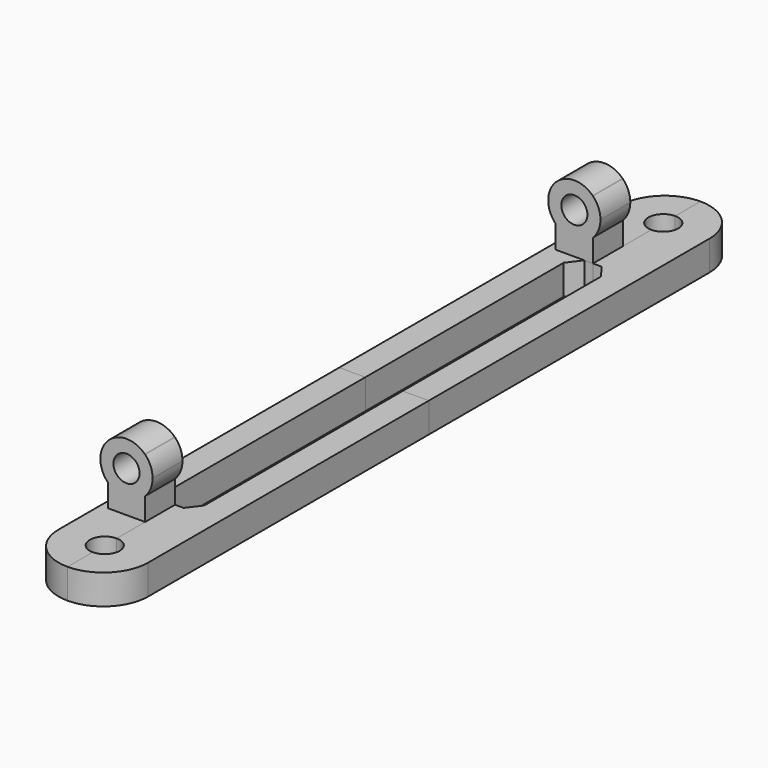
from build123d import *

# Parameters (mm, degrees)
F1_DEPTH = 4
F3_START = -35
F2_R     = 1.75
F3_DEPTH = 5
F6_R     = 5.99999
F6_2_R   = 5.99999
F6_3_R   = 5.99999
F6_4_R   = 5.99999


# Not quite as in the source:
# - a fillet or chamfer is up to 0.001 mm smaller than in the source, because OpenCascade refuses the exact size


with BuildPart() as f1:
    # F0 (on Top) → F1 (new body)
    with BuildSketch(Plane.XY):
        with BuildLine():
            Line((-6, 0), (-2.5, 0))
            Line((-2.5, 0), (-2.5, 33.2198664546))
            Line((-2.5, 33.2198664546), (-1.1564682936, 35))
            Line((-1.1564682936, 35), (0, 35))
            Line((0, 35), (0, 44.77))
            ThreePointArc((0, 44.77), (-2, 46.77), (0, 48.77))
            Line((0, 48.77), (0, 53))
            Line((0, 53), (-6, 53))
            Line((-6, 53), (-6, 0))
        make_face()
    extrude(amount=F1_DEPTH)


with BuildPart() as f3:
    # F2 (on Front) → F3 (new body)
    with BuildSketch(Plane.XZ.offset(F3_START)):
        with BuildLine():
            ThreePointArc((-5, 7.0505102572), (-2.5, 6), (0, 7.0505102572))
            Line((0, 7.0505102572), (0, 11.9494897428))
            ThreePointArc((0, 11.9494897428), (-0.0251262658, 11.9748737342), (-0.0505102572, 12))
            Line((-0.0505102572, 12), (-4.9494897428, 12))
            ThreePointArc((-4.9494897428, 12), (-4.9748737342, 11.9748737342), (-5, 11.9494897428))
            Line((-5, 11.9494897428), (-5, 7.0505102572))
        make_face()
        with Locations((-2.5, 9.5)):
            Circle(F2_R, mode=Mode.SUBTRACT)
        with BuildLine():
            Line((-5, 4), (0, 4))
            Line((0, 4), (0, 7.0505102572))
            ThreePointArc((0, 7.0505102572), (-2.5, 6), (-5, 7.0505102572))
            Line((-5, 7.0505102572), (-5, 4))
        make_face()
        with BuildLine():
            Line((0, 11.9494897428), (0, 7.0505102572))
            ThreePointArc((0, 7.0505102572), (0.7403703492, 8.1771243445), (1, 9.5))
            ThreePointArc((1, 9.5), (0.7403703492, 10.8228756555), (0, 11.9494897428))
        make_face()
        with BuildLine():
            Line((-4.9494897428, 12), (-0.0505102572, 12))
            ThreePointArc((-0.0505102572, 12), (-2.5, 13), (-4.9494897428, 12))
        make_face()
        with BuildLine():
            ThreePointArc((-5, 11.9494897428), (-6, 9.5), (-5, 7.0505102572))
            Line((-5, 7.0505102572), (-5, 11.9494897428))
        make_face()
    extrude(amount=-F3_DEPTH)


with BuildPart() as f4_1:
    # F4: instance of F1
    add(f1.part.mirror(Plane(origin=(-4.25, 0, 2), x_dir=(1, 0, 0), z_dir=(0, -1, 0))))


with BuildPart() as f4_2:
    # F4: instance of F3
    add(f3.part.mirror(Plane(origin=(-4.25, 0, 2), x_dir=(1, 0, 0), z_dir=(0, -1, 0))))


with BuildPart() as f5_1:
    # F5: instance of F1
    add(f1.part.mirror(Plane(origin=(0, -39.885, 2), x_dir=(0, 1, 0), z_dir=(1, 0, 0))))

    # F6#3 (radius 6 in the source; OpenCascade refuses exactly that, so slightly less here)
    f6_3_edges = [f5_1.edges().sort_by_distance(p)[0] for p in [
        (6, 53, 2),
    ]]
    fillet(f6_3_edges, radius=F6_3_R)


with BuildPart() as f5_2:
    # F5: instance of F4_1
    add(f4_1.part.mirror(Plane(origin=(0, -39.885, 2), x_dir=(0, 1, 0), z_dir=(1, 0, 0))))

    # F6 (radius 6 in the source; OpenCascade refuses exactly that, so slightly less here)
    f6_edges = [f5_2.edges().sort_by_distance(p)[0] for p in [
        (6, -53, 2),
    ]]
    fillet(f6_edges, radius=F6_R)


with BuildPart() as f4_1_1:
    add(f4_1.part)

    # F6#2 (radius 6 in the source; OpenCascade refuses exactly that, so slightly less here)
    f6_2_edges = [f4_1_1.edges().sort_by_distance(p)[0] for p in [
        (-6, -53, 2),
    ]]
    fillet(f6_2_edges, radius=F6_2_R)


with BuildPart() as f1_1:
    add(f1.part)

    # F6#4 (radius 6 in the source; OpenCascade refuses exactly that, so slightly less here)
    f6_4_edges = [f1_1.edges().sort_by_distance(p)[0] for p in [
        (-6, 53, 2),
    ]]
    fillet(f6_4_edges, radius=F6_4_R)


solid = Compound([f3.part, f4_2.part, f5_1.part, f5_2.part, f4_1_1.part, f1_1.part])
